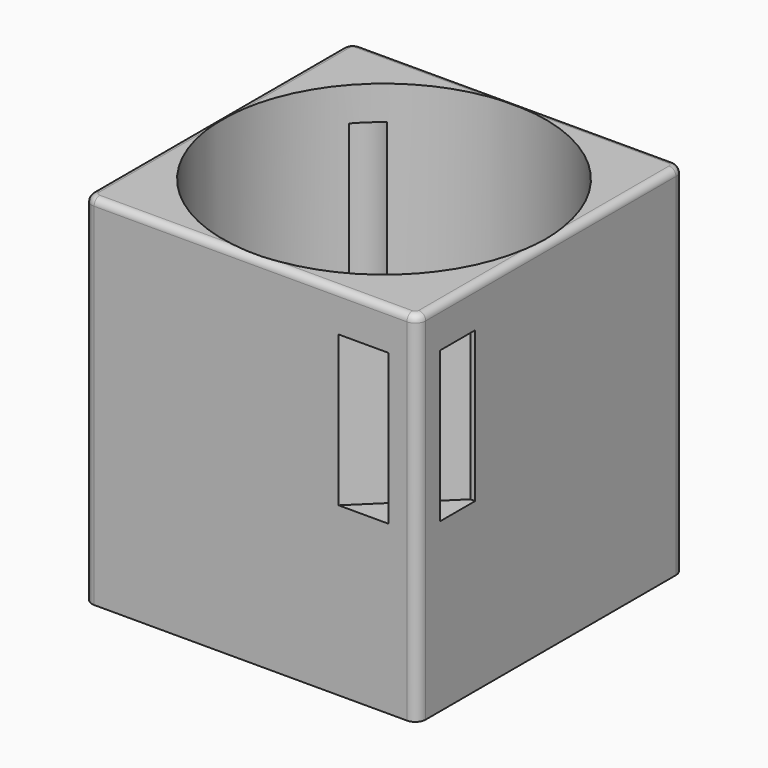
from build123d import *

# Parameters (mm, degrees)
F0_W         = 96
F0_H         = 96
F1_DEPTH     = 103
F2_R         = 16.5
F3_DEPTH     = 100
F4_R         = 46.5
F5_DEPTH     = 80
F6_T1_DEPTH  = 106
F6_T3_DEPTH  = 106
F7_T1_DEPTH  = 110.4999999999
F7_T4_ANGLE  = 90
F7_T6_ANGLE  = 90
F7_T8_ANGLE  = 90
F7_T10_ANGLE = 90
F9_SIZE      = 2
F8_W         = 14.3129900098
F8_H         = 43.2826243341
F12_R        = 5
F13_W        = 11.0455658287
F13_H        = 45.8308011293


# Not quite as in the source:
# - a fillet or chamfer that OpenCascade refuses, or shapes differently, is made with other operations: its cross-section is extruded or revolved along the edge and cut away or added


with BuildPart() as f1:
    # F0 (on Top) → F1 (new body)
    with BuildSketch(Plane.XY):
        Rectangle(F0_W, F0_H)
    extrude(amount=F1_DEPTH)

    # F2 (on face) → F3 (cut)
    with BuildSketch(Plane.XY.offset(103)):
        Circle(F2_R)
    extrude(amount=-F3_DEPTH, mode=Mode.SUBTRACT)

    # F4 (on face) → F5 (cut)
    with BuildSketch(Plane.XY.offset(103)):
        Circle(F4_R)
    extrude(amount=-F5_DEPTH, mode=Mode.SUBTRACT)

    # F6: fillet of radius 2 on 4 edges, made by hand

    # F6_s2 → F6_t1 (cut)
    with BuildSketch(Plane.YZ.offset(-53)):
        with BuildLine():
            ThreePointArc((48, 101), (47.4142135624, 102.4142135624), (46, 103))
            Line((46, 103), (48, 103))
            Line((48, 103), (48, 101))
        make_face()
        with BuildLine():
            ThreePointArc((-48, 101), (-47.4142135624, 102.4142135624), (-46, 103))
            Line((-46, 103), (-48, 103))
            Line((-48, 103), (-48, 101))
        make_face()
    extrude(amount=F6_T1_DEPTH, mode=Mode.SUBTRACT)

    # F6_s4 → F6_t3 (cut)
    with BuildSketch(Plane.XZ.offset(-53)):
        with BuildLine():
            ThreePointArc((48, 101), (47.4142135624, 102.4142135624), (46, 103))
            Line((46, 103), (48, 103))
            Line((48, 103), (48, 101))
        make_face()
        with BuildLine():
            ThreePointArc((-46, 103), (-47.4142135624, 102.4142135624), (-48, 101))
            Line((-48, 101), (-48, 103))
            Line((-48, 103), (-46, 103))
        make_face()
    extrude(amount=F6_T3_DEPTH, mode=Mode.SUBTRACT)

    # F7: fillet of radius 3 on 4 edges, made by hand

    # F7_s2 → F7_t1 (cut)
    with BuildSketch(Plane.XY.offset(-7.5)):
        with BuildLine():
            ThreePointArc((48, -45), (47.1213203436, -47.1213203436), (45, -48))
            Line((45, -48), (48, -48))
            Line((48, -48), (48, -45))
        make_face()
        with BuildLine():
            ThreePointArc((-45, -48), (-47.1213203436, -47.1213203436), (-48, -45))
            Line((-48, -45), (-48, -48))
            Line((-48, -48), (-45, -48))
        make_face()
        with BuildLine():
            ThreePointArc((-45, 48), (-47.1213203436, 47.1213203436), (-48, 45))
            Line((-48, 45), (-48, 48))
            Line((-48, 48), (-45, 48))
        make_face()
        with BuildLine():
            ThreePointArc((48, 45), (47.1213203436, 47.1213203436), (45, 48))
            Line((45, 48), (48, 48))
            Line((48, 48), (48, 45))
        make_face()
    extrude(amount=F7_T1_DEPTH, mode=Mode.SUBTRACT)

    # F7_s3 → F7_t4 (revolve, cut)
    with BuildSketch(Plane.XZ.offset(-45)):
        with BuildLine():
            ThreePointArc((46.0000000001, 103), (47.4142135624, 102.4142135624), (48, 101.0000000001))
            Line((48, 101.0000000001), (48, 103))
            Line((48, 103), (46.0000000001, 103))
        make_face()
    revolve(axis=Axis((45, 45, 103), (0, 0, 1)), revolution_arc=F7_T4_ANGLE, mode=Mode.SUBTRACT)

    # F7_s5 → F7_t6 (revolve, cut)
    with BuildSketch(Plane.YZ.offset(-45)):
        with BuildLine():
            ThreePointArc((46.0000000001, 103), (47.4142135624, 102.4142135624), (48, 101.0000000001))
            Line((48, 101.0000000001), (48, 103))
            Line((48, 103), (46.0000000001, 103))
        make_face()
    revolve(axis=Axis((-45, 45, 103), (0, 0, 1)), revolution_arc=F7_T6_ANGLE, mode=Mode.SUBTRACT)

    # F7_s7 → F7_t8 (revolve, cut)
    with BuildSketch(Plane.XZ.offset(45)):
        with BuildLine():
            ThreePointArc((-46.0000000001, 103), (-47.4142135624, 102.4142135624), (-48, 101.0000000001))
            Line((-48, 101.0000000001), (-48, 103))
            Line((-48, 103), (-46.0000000001, 103))
        make_face()
    revolve(axis=Axis((-45, -45, 103), (0, 0, 1)), revolution_arc=F7_T8_ANGLE, mode=Mode.SUBTRACT)

    # F7_s9 → F7_t10 (revolve, cut)
    with BuildSketch(Plane.YZ.offset(45)):
        with BuildLine():
            ThreePointArc((-46.0000000001, 103), (-47.4142135624, 102.4142135624), (-48, 101.0000000001))
            Line((-48, 101.0000000001), (-48, 103))
            Line((-48, 103), (-46.0000000001, 103))
        make_face()
    revolve(axis=Axis((45, -45, 103), (0, 0, 1)), revolution_arc=F7_T10_ANGLE, mode=Mode.SUBTRACT)

    # F9
    f9_edges = [f1.edges().sort_by_distance(p)[0] for p in [
        (-16.5, 0, 23),
    ]]
    chamfer(f9_edges, length=F9_SIZE)

    # F11: sweep along a path in F10
    with BuildLine(Plane.XY.offset(23)) as f11_path:
        Line((27.1213203436, -47.9204392359), (48.4205447137, -27.1213203436))
    # F8 (on face) → F11 (sweep, cut)
    with BuildSketch(Plane.XZ.offset(48)):
        with Locations((32.499153167, 69.7716791183)):
            Rectangle(F8_W, F8_H)
    sweep(path=f11_path.line, mode=Mode.SUBTRACT)

    # F12
    f12_edges = [f1.edges().sort_by_distance(p)[0] for p in [
        (-46.5, 0, 23),
    ]]
    fillet(f12_edges, radius=F12_R)

    # F13 (on face) → F14 (revolve, cut)
    with BuildSketch(Plane(origin=(-48, 0, 0), x_dir=(0, -1, 0), z_dir=(-1, 0, 0))):
        with Locations((-33.7943071499, 70.3311860561)):
            Rectangle(F13_W, F13_H)
    revolve(axis=Axis((-45, 48, 50.5), (0, 0, -1)), mode=Mode.SUBTRACT)


solid = f1.part
